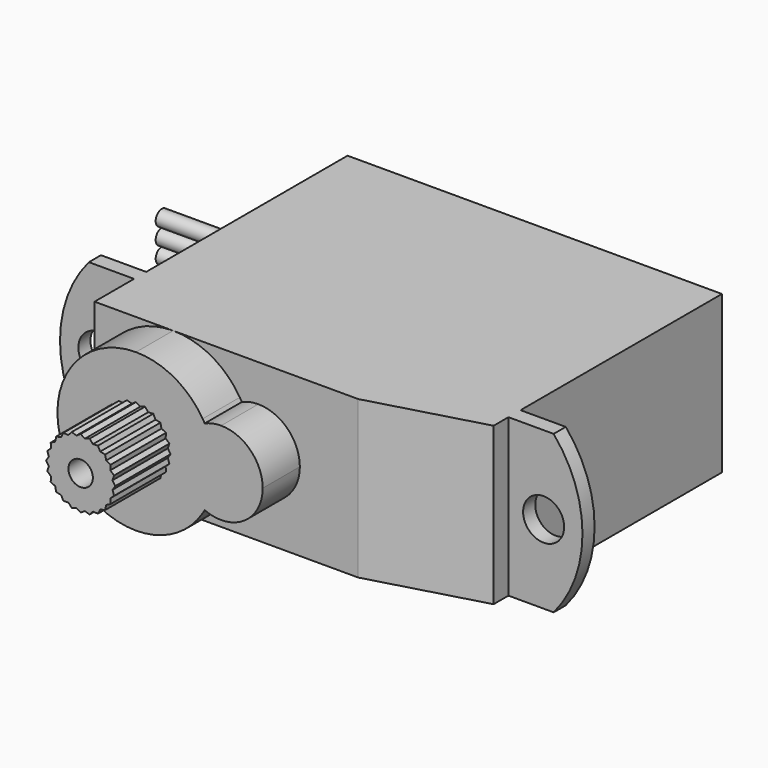
from build123d import *

# Parameters (mm, degrees)
F0_W      = 19.4564
F0_H      = 8.1661
F1_DEPTH  = 16.4338
F3_DEPTH  = 8.1661
F5_DEPTH  = 2.413
F6_R      = 0.635
F7_DEPTH  = 3.5941
F9_R      = 1.0668
F10_DEPTH = 0.7874
F11_R     = 0.40005
F12_DEPTH = 6.35


# Not quite as in the source:
# - a pattern or mirror of a feature is missing from the dataset's text; its kind, count and spacing are read off the source's solid


with BuildPart() as f1:
    # F0 (on Front) → F1 (new body)
    with BuildSketch(Plane.XZ):
        Rectangle(F0_W, F0_H)
    extrude(amount=F1_DEPTH)

    # F2 (on face) → F3 (cut, through all)
    with BuildSketch(Plane(origin=(0, 0, -4.08305), x_dir=(1, 0, 0), z_dir=(0, 0, -1))):
        Polygon((3.9751, 16.4338), (9.7282, 14.8336), (9.7282, 16.4338), align=None)
    extrude(amount=-F3_DEPTH, mode=Mode.SUBTRACT)

    # F4 (on face) → F5 (join)
    with BuildSketch(Plane.XZ.offset(16.4338)):
        with BuildLine():
            ThreePointArc((-2.0754022956, -1.9819683724), (-3.3782, 0), (-2.0754022956, 1.9819683724))
            ThreePointArc((-2.0754022956, 1.9819683724), (-2.1263891254, 2.071139592), (-2.1796029577, 2.159))
            ThreePointArc((-2.1796029577, 2.159), (-3.6632327094, 3.5697760652), (-5.6451500171, 4.08305))
            ThreePointArc((-5.6451500171, 4.08305), (-8.532302349, 2.8871523369), (-9.7282, 0))
            ThreePointArc((-9.7282, 0), (-8.5323023429, -2.8871523429), (-5.64515, -4.08305))
            ThreePointArc((-5.64515, -4.08305), (-3.663232702, -3.5697760611), (-2.1796029577, -2.159))
            ThreePointArc((-2.1796029577, -2.159), (-2.1263891254, -2.071139592), (-2.0754022956, -1.9819683724))
        make_face()
        with BuildLine():
            ThreePointArc((-2.0754022956, -1.9819683724), (-1.6925081197, -1.023679378), (-1.5621, 0))
            ThreePointArc((-1.5621, 0), (-1.6925081197, 1.023679378), (-2.0754022956, 1.9819683724))
            ThreePointArc((-2.0754022956, 1.9819683724), (-3.3782, 0), (-2.0754022956, -1.9819683724))
        make_face()
        with BuildLine():
            ThreePointArc((-2.0754022956, 1.9819683724), (-1.6925081197, 1.023679378), (-1.5621, 0))
            ThreePointArc((-1.5621, 0), (-1.6925081197, -1.023679378), (-2.0754022956, -1.9819683724))
            ThreePointArc((-2.0754022956, -1.9819683724), (-1.656356313, -2.1142789215), (-1.2192, -2.159))
            ThreePointArc((-1.2192, -2.159), (0.3074435406, -1.5266435406), (0.9398, 0))
            ThreePointArc((0.9398, 0), (0.3074435406, 1.5266435406), (-1.2192, 2.159))
            ThreePointArc((-1.2192, 2.159), (-1.656356313, 2.1142789215), (-2.0754022956, 1.9819683724))
        make_face()
    extrude(amount=F5_DEPTH)

    # F6 (on face) → F7 (join)
    with BuildSketch(Plane.XZ.offset(18.8468)):
        Polygon((-5.4271647327, 1.6557624907), (-5.64515, 1.79705), (-5.8631352673, 1.6557624907), (-6.110260765, 1.7358170061), (-6.2842504662, 1.5429250133), (-6.543675, 1.5562909519), (-6.6618120245, 1.324939746), (-6.9158562411, 1.2707062411), (-6.970089746, 1.0166620245), (-7.2014409519, 0.898525), (-7.1880750133, 0.6391004662), (-7.3809670061, 0.465110765), (-7.3009124907, 0.2179852673), (-7.4422, 0), (-7.3009124907, -0.2179852673), (-7.3809670061, -0.465110765), (-7.1880750133, -0.6391004662), (-7.2014409519, -0.898525), (-6.970089746, -1.0166620245), (-6.9158562411, -1.2707062411), (-6.6618120245, -1.324939746), (-6.543675, -1.5562909519), (-6.2842504662, -1.5429250133), (-6.110260765, -1.7358170061), (-5.8631352673, -1.6557624907), (-5.64515, -1.79705), (-5.4271647327, -1.6557624907), (-5.180039235, -1.7358170061), (-5.0060495338, -1.5429250133), (-4.746625, -1.5562909519), (-4.6284879755, -1.324939746), (-4.3744437589, -1.2707062411), (-4.320210254, -1.0166620245), (-4.0888590481, -0.898525), (-4.1022249867, -0.6391004662), (-3.9093329939, -0.465110765), (-3.9893875093, -0.2179852673), (-3.8481, 0), (-3.9893875093, 0.2179852673), (-3.9093329939, 0.465110765), (-4.1022249867, 0.6391004662), (-4.0888590481, 0.898525), (-4.320210254, 1.0166620245), (-4.3744437589, 1.2707062411), (-4.6284879755, 1.324939746), (-4.746625, 1.5562909519), (-5.0060495338, 1.5429250133), (-5.180039235, 1.7358170061), align=None)
        with Locations((-5.64515, 0)):
            Circle(F6_R, mode=Mode.SUBTRACT)
    extrude(amount=F7_DEPTH)

    # F9 (on offset) → F10 (join)
    with BuildSketch(Plane.XZ.offset(13.081)):
        with BuildLine():
            Line((12.0777, 4.08305), (9.7282, 4.08305))
            Line((9.7282, 4.08305), (9.7282, -4.08305))
            Line((9.7282, -4.08305), (12.0777, -4.08305))
            ThreePointArc((12.0777, -4.08305), (13.5763, 0), (12.0777, 4.08305))
        make_face()
        with Locations((11.557, 0)):
            Circle(F9_R, mode=Mode.SUBTRACT)
    f10 = extrude(amount=F10_DEPTH)

    # F10_copies: F10 across plane
    add(f10.mirror(Plane(origin=(0, 0, 0), x_dir=(0, 0, -1), z_dir=(-1, 0, 0))))

    # F11 (on face) → F12 (join)
    with BuildSketch(Plane(origin=(-9.7282, 0, 0), x_dir=(0, -1, 0), z_dir=(-1, 0, 0))):
        with Locations((4.1275, 0.8636)):
            Circle(F11_R)
        with Locations((4.1275, 0)):
            Circle(F11_R)
        with Locations((4.1275, -0.8636)):
            Circle(F11_R)
    extrude(amount=F12_DEPTH)


solid = f1.part
